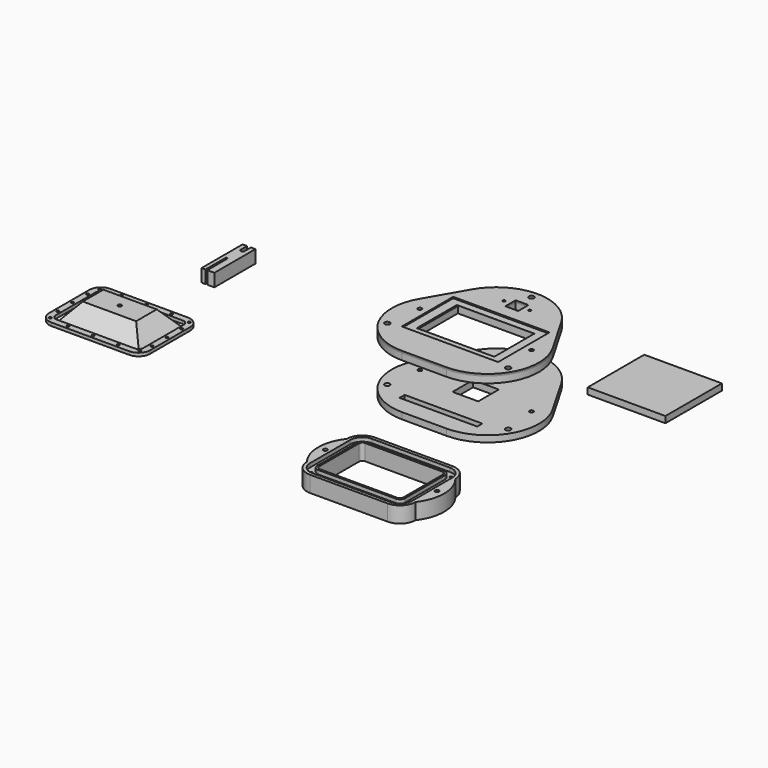
from build123d import *

# Parameters (mm, degrees)
F0_R            = 4
F0_R_2          = 3
F0_W            = 150
F0_H            = 100
F0_R_3          = 2
F0_W_2          = 20
F0_H_2          = 20
F0_W_3          = 1.5
F0_H_3          = 78
F1_DEPTH        = 10
F2_DEPTH        = 1
F3_START        = 1
F3_DEPTH        = 2
F0_W_4          = 121
F0_H_4          = 110
F4_DEPTH        = 10
F6_DEPTH        = 25
F7_DEPTH        = 6
F8_D            = 4
F9_DEPTH        = 5
F10_D           = 4
F10_CSINK_D     = 8
F10_CSINK_ANGLE = 90
F11_DEPTH       = 25
F0_W_5          = 118
F12_DEPTH       = 10
F14_W           = 40
F14_H           = 40
F14_W_2         = 121
F14_H_2         = 10
F15_DEPTH       = 25
F0_W_6          = 125
F0_H_5          = 82
F16_DEPTH       = 25
F16_TAPER       = 40
F18_D           = 6
F18_DEPTH       = 10
F18_TIP         = 1.8025818571
F19_DEPTH       = 20


with BuildPart() as f1:
    # F0 (on Top) → F1 (new body)
    with BuildSketch(Plane.XY):
        with BuildLine():
            Line((-34.6410161514, -100), (34.6410161514, -100))
            ThreePointArc((34.6410161514, -100), (103.9230484541, -60), (103.9230484541, 20))
            Line((103.9230484541, 20), (69.2820323028, 80))
            ThreePointArc((69.2820323028, 80), (0, 120), (-69.2820323028, 80))
            Line((-69.2820323028, 80), (-103.9230484541, 20))
            ThreePointArc((-103.9230484541, 20), (-103.9230484541, -60), (-34.6410161514, -100))
        make_face()
        with Locations((-94.1006406596, -54.3290302157)):
            Circle(F0_R, mode=Mode.SUBTRACT)
        with Locations((-87, 0)):
            Circle(F0_R_2, mode=Mode.SUBTRACT)
        with Locations((94.1006406596, -54.3290302157)):
            Circle(F0_R, mode=Mode.SUBTRACT)
        Rectangle(F0_W, F0_H, mode=Mode.SUBTRACT)
        with Locations((87, 0)):
            Circle(F0_R_2, mode=Mode.SUBTRACT)
        with Locations((-20, 80.2838653326)):
            Circle(F0_R_3, mode=Mode.SUBTRACT)
        with Locations((0, 80.2838653326)):
            Rectangle(F0_W_2, F0_H_2, mode=Mode.SUBTRACT)
        with Locations((20, 80.2838653326)):
            Circle(F0_R_3, mode=Mode.SUBTRACT)
        with Locations((0, 108.6580604315)):
            Circle(F0_R, mode=Mode.SUBTRACT)
        Rectangle(F0_W, F0_H)
        Polygon((-60.5, -39), (-60.5, 39), (-59, 39), (59, 39), (60.5, 39), (60.5, -39), (59, -39), (-59, -39), align=None, mode=Mode.SUBTRACT)
        with Locations((-59.75, 0)):
            Rectangle(F0_W_3, F0_H_3)
        with Locations((59.75, 0)):
            Rectangle(F0_W_3, F0_H_3)
    extrude(amount=-F1_DEPTH)

    # F5 (on face) → F11 (cut)
    with BuildSketch(Plane(origin=(0, 0, -10), x_dir=(1, 0, 0), z_dir=(0, 0, -1))):
        Polygon((60.5, 62.5), (60.5, 72.5), (-60.5, 72.5), (-60.5, 62.5), (-60.5, 39), (-59, 39), (59, 39), (60.5, 39), align=None)
    extrude(amount=-F11_DEPTH, mode=Mode.SUBTRACT)


with BuildPart() as f2:
    # F0 (on Top) → F2 (new body)
    with BuildSketch(Plane.XY):
        with BuildLine():
            Line((-34.6410161514, -100), (34.6410161514, -100))
            ThreePointArc((34.6410161514, -100), (103.9230484541, -60), (103.9230484541, 20))
            Line((103.9230484541, 20), (69.2820323028, 80))
            ThreePointArc((69.2820323028, 80), (0, 120), (-69.2820323028, 80))
            Line((-69.2820323028, 80), (-103.9230484541, 20))
            ThreePointArc((-103.9230484541, 20), (-103.9230484541, -60), (-34.6410161514, -100))
        make_face()
        with Locations((-94.1006406596, -54.3290302157)):
            Circle(F0_R, mode=Mode.SUBTRACT)
        with Locations((-87, 0)):
            Circle(F0_R_2, mode=Mode.SUBTRACT)
        with Locations((94.1006406596, -54.3290302157)):
            Circle(F0_R, mode=Mode.SUBTRACT)
        Rectangle(F0_W, F0_H, mode=Mode.SUBTRACT)
        with Locations((87, 0)):
            Circle(F0_R_2, mode=Mode.SUBTRACT)
        with Locations((-20, 80.2838653326)):
            Circle(F0_R_3, mode=Mode.SUBTRACT)
        with Locations((0, 80.2838653326)):
            Rectangle(F0_W_2, F0_H_2, mode=Mode.SUBTRACT)
        with Locations((20, 80.2838653326)):
            Circle(F0_R_3, mode=Mode.SUBTRACT)
        with Locations((0, 108.6580604315)):
            Circle(F0_R, mode=Mode.SUBTRACT)
        Rectangle(F0_W, F0_H)
        Polygon((-60.5, -39), (-60.5, 39), (-59, 39), (59, 39), (60.5, 39), (60.5, -39), (59, -39), (-59, -39), align=None, mode=Mode.SUBTRACT)
    extrude(amount=F2_DEPTH)


with BuildPart() as f3:
    # F0 (on Top) → F3 (new body)
    with BuildSketch(Plane.XY.offset(F3_START)):
        with BuildLine():
            Line((-34.6410161514, -100), (34.6410161514, -100))
            ThreePointArc((34.6410161514, -100), (103.9230484541, -60), (103.9230484541, 20))
            Line((103.9230484541, 20), (69.2820323028, 80))
            ThreePointArc((69.2820323028, 80), (0, 120), (-69.2820323028, 80))
            Line((-69.2820323028, 80), (-103.9230484541, 20))
            ThreePointArc((-103.9230484541, 20), (-103.9230484541, -60), (-34.6410161514, -100))
        make_face()
        with Locations((-94.1006406596, -54.3290302157)):
            Circle(F0_R, mode=Mode.SUBTRACT)
        with Locations((-87, 0)):
            Circle(F0_R_2, mode=Mode.SUBTRACT)
        with Locations((94.1006406596, -54.3290302157)):
            Circle(F0_R, mode=Mode.SUBTRACT)
        Rectangle(F0_W, F0_H, mode=Mode.SUBTRACT)
        with Locations((87, 0)):
            Circle(F0_R_2, mode=Mode.SUBTRACT)
        with Locations((-20, 80.2838653326)):
            Circle(F0_R_3, mode=Mode.SUBTRACT)
        with Locations((0, 80.2838653326)):
            Rectangle(F0_W_2, F0_H_2, mode=Mode.SUBTRACT)
        with Locations((20, 80.2838653326)):
            Circle(F0_R_3, mode=Mode.SUBTRACT)
        with Locations((0, 108.6580604315)):
            Circle(F0_R, mode=Mode.SUBTRACT)
    extrude(amount=F3_DEPTH)


with BuildPart() as f4:
    # F0 (on Top) → F4 (new body)
    with BuildSketch(Plane.XY):
        with Locations((270.5340873003, 10.6164294481)):
            Rectangle(F0_W_4, F0_H_4)
    extrude(amount=F4_DEPTH)


with BuildPart() as f6:
    # F0 (on Top) → F6 (new body)
    with BuildSketch(Plane.XY):
        with BuildLine():
            ThreePointArc((223.1106657982, -358.8882369786), (222.6106657982, -357.2299245834), (223.1106657982, -355.5716121883))
            Line((223.1106657982, -355.5716121883), (223.1106657982, -318.2299245834))
            ThreePointArc((223.1106657982, -318.2299245834), (216.0812285467, -301.259361835), (199.1106657982, -294.2299245834))
            Line((199.1106657982, -294.2299245834), (78.1106657982, -294.2299245834))
            ThreePointArc((78.1106657982, -294.2299245834), (61.1401030497, -301.259361835), (54.1106657982, -318.2299245834))
            Line((54.1106657982, -318.2299245834), (54.1106657982, -355.5716121883))
            ThreePointArc((54.1106657982, -355.5716121883), (54.4829471215, -356.3638991797), (54.6106657982, -357.2299245834))
            ThreePointArc((54.6106657982, -357.2299245834), (54.4829471215, -358.0959499872), (54.1106657982, -358.8882369786))
            Line((54.1106657982, -358.8882369786), (54.1106657982, -396.2299245834))
            ThreePointArc((54.1106657982, -396.2299245834), (61.1401030497, -413.2004873319), (78.1106657982, -420.2299245834))
            Line((78.1106657982, -420.2299245834), (199.1106657982, -420.2299245834))
            ThreePointArc((199.1106657982, -420.2299245834), (216.0812285467, -413.2004873319), (223.1106657982, -396.2299245834))
            Line((223.1106657982, -396.2299245834), (223.1106657982, -358.8882369786))
        make_face()
        with BuildLine():
            ThreePointArc((59.1106657982, -318.2299245834), (64.6756369556, -304.7948957409), (78.1106657982, -299.2299245834))
            Line((78.1106657982, -299.2299245834), (199.1106657982, -299.2299245834))
            ThreePointArc((199.1106657982, -299.2299245834), (212.5456946407, -304.7948957409), (218.1106657982, -318.2299245834))
            Line((218.1106657982, -318.2299245834), (218.1106657982, -396.2299245834))
            ThreePointArc((218.1106657982, -396.2299245834), (212.5456946407, -409.664953426), (199.1106657982, -415.2299245834))
            Line((199.1106657982, -415.2299245834), (78.1106657982, -415.2299245834))
            ThreePointArc((78.1106657982, -415.2299245834), (64.6756369556, -409.664953426), (59.1106657982, -396.2299245834))
            Line((59.1106657982, -396.2299245834), (59.1106657982, -318.2299245834))
        make_face(mode=Mode.SUBTRACT)
        with BuildLine():
            Line((199.1106657982, -299.2299245834), (78.1106657982, -299.2299245834))
            ThreePointArc((78.1106657982, -299.2299245834), (64.6756369556, -304.7948957409), (59.1106657982, -318.2299245834))
            Line((59.1106657982, -318.2299245834), (59.1106657982, -396.2299245834))
            ThreePointArc((59.1106657982, -396.2299245834), (64.6756369556, -409.664953426), (78.1106657982, -415.2299245834))
            Line((78.1106657982, -415.2299245834), (199.1106657982, -415.2299245834))
            ThreePointArc((199.1106657982, -415.2299245834), (212.5456946407, -409.664953426), (218.1106657982, -396.2299245834))
            Line((218.1106657982, -396.2299245834), (218.1106657982, -318.2299245834))
            ThreePointArc((218.1106657982, -318.2299245834), (212.5456946407, -304.7948957409), (199.1106657982, -299.2299245834))
        make_face()
        with BuildLine():
            ThreePointArc((70.1106657982, -318.2299245834), (72.4538115487, -312.5730703339), (78.1106657982, -310.2299245834))
            Line((78.1106657982, -310.2299245834), (199.1106657982, -310.2299245834))
            ThreePointArc((199.1106657982, -310.2299245834), (204.7675200477, -312.5730703339), (207.1106657982, -318.2299245834))
            Line((207.1106657982, -318.2299245834), (207.1106657982, -396.2299245834))
            ThreePointArc((207.1106657982, -396.2299245834), (204.7675200477, -401.8867788329), (199.1106657982, -404.2299245834))
            Line((199.1106657982, -404.2299245834), (78.1106657982, -404.2299245834))
            ThreePointArc((78.1106657982, -404.2299245834), (72.4538115487, -401.8867788329), (70.1106657982, -396.2299245834))
            Line((70.1106657982, -396.2299245834), (70.1106657982, -318.2299245834))
        make_face(mode=Mode.SUBTRACT)
        with BuildLine():
            Line((199.1106657982, -310.2299245834), (78.1106657982, -310.2299245834))
            ThreePointArc((78.1106657982, -310.2299245834), (72.4538115487, -312.5730703339), (70.1106657982, -318.2299245834))
            Line((70.1106657982, -318.2299245834), (70.1106657982, -396.2299245834))
            ThreePointArc((70.1106657982, -396.2299245834), (72.4538115487, -401.8867788329), (78.1106657982, -404.2299245834))
            Line((78.1106657982, -404.2299245834), (199.1106657982, -404.2299245834))
            ThreePointArc((199.1106657982, -404.2299245834), (204.7675200477, -401.8867788329), (207.1106657982, -396.2299245834))
            Line((207.1106657982, -396.2299245834), (207.1106657982, -318.2299245834))
            ThreePointArc((207.1106657982, -318.2299245834), (204.7675200477, -312.5730703339), (199.1106657982, -310.2299245834))
        make_face()
        with BuildLine():
            ThreePointArc((73.1106657982, -318.2299245834), (74.5751318923, -314.6943906775), (78.1106657982, -313.2299245834))
            Line((78.1106657982, -313.2299245834), (199.1106657982, -313.2299245834))
            ThreePointArc((199.1106657982, -313.2299245834), (202.6461997041, -314.6943906775), (204.1106657982, -318.2299245834))
            Line((204.1106657982, -318.2299245834), (204.1106657982, -396.2299245834))
            ThreePointArc((204.1106657982, -396.2299245834), (202.6461997041, -399.7654584894), (199.1106657982, -401.2299245834))
            Line((199.1106657982, -401.2299245834), (78.1106657982, -401.2299245834))
            ThreePointArc((78.1106657982, -401.2299245834), (74.5751318923, -399.7654584894), (73.1106657982, -396.2299245834))
            Line((73.1106657982, -396.2299245834), (73.1106657982, -318.2299245834))
        make_face(mode=Mode.SUBTRACT)
        with BuildLine():
            Line((54.1106657982, -355.5716121883), (54.1106657982, -318.2299245834))
            ThreePointArc((54.1106657982, -318.2299245834), (40.659391154, -357.2299245834), (54.1106657982, -396.2299245834))
            Line((54.1106657982, -396.2299245834), (54.1106657982, -358.8882369786))
            ThreePointArc((54.1106657982, -358.8882369786), (48.6106657982, -357.2299245834), (54.1106657982, -355.5716121883))
        make_face()
        with BuildLine():
            ThreePointArc((223.1106657982, -355.5716121883), (226.476691202, -354.3576432602), (228.6106657982, -357.2299245834))
            ThreePointArc((228.6106657982, -357.2299245834), (226.476691202, -360.1022059067), (223.1106657982, -358.8882369786))
            Line((223.1106657982, -358.8882369786), (223.1106657982, -396.2299245834))
            ThreePointArc((223.1106657982, -396.2299245834), (236.5619404423, -357.2299245834), (223.1106657982, -318.2299245834))
            Line((223.1106657982, -318.2299245834), (223.1106657982, -355.5716121883))
        make_face()
    extrude(amount=-F6_DEPTH)

    # F0 (on Top) → F7 (cut)
    with BuildSketch(Plane.XY):
        with BuildLine():
            Line((199.1106657982, -299.2299245834), (78.1106657982, -299.2299245834))
            ThreePointArc((78.1106657982, -299.2299245834), (64.6756369556, -304.7948957409), (59.1106657982, -318.2299245834))
            Line((59.1106657982, -318.2299245834), (59.1106657982, -396.2299245834))
            ThreePointArc((59.1106657982, -396.2299245834), (64.6756369556, -409.664953426), (78.1106657982, -415.2299245834))
            Line((78.1106657982, -415.2299245834), (199.1106657982, -415.2299245834))
            ThreePointArc((199.1106657982, -415.2299245834), (212.5456946407, -409.664953426), (218.1106657982, -396.2299245834))
            Line((218.1106657982, -396.2299245834), (218.1106657982, -318.2299245834))
            ThreePointArc((218.1106657982, -318.2299245834), (212.5456946407, -304.7948957409), (199.1106657982, -299.2299245834))
        make_face()
        with BuildLine():
            ThreePointArc((70.1106657982, -318.2299245834), (72.4538115487, -312.5730703339), (78.1106657982, -310.2299245834))
            Line((78.1106657982, -310.2299245834), (199.1106657982, -310.2299245834))
            ThreePointArc((199.1106657982, -310.2299245834), (204.7675200477, -312.5730703339), (207.1106657982, -318.2299245834))
            Line((207.1106657982, -318.2299245834), (207.1106657982, -396.2299245834))
            ThreePointArc((207.1106657982, -396.2299245834), (204.7675200477, -401.8867788329), (199.1106657982, -404.2299245834))
            Line((199.1106657982, -404.2299245834), (78.1106657982, -404.2299245834))
            ThreePointArc((78.1106657982, -404.2299245834), (72.4538115487, -401.8867788329), (70.1106657982, -396.2299245834))
            Line((70.1106657982, -396.2299245834), (70.1106657982, -318.2299245834))
        make_face(mode=Mode.SUBTRACT)
    extrude(amount=-F7_DEPTH, mode=Mode.SUBTRACT)

    # F8 (through all)
    with Locations(Plane.XY):
        with Locations((68.5647242522, -308.6839830374), (99.5444750786, -304.7299245834), (138.6106657982, -304.7299245834), (177.6768565178, -304.7299245834), (208.6566073442, -308.6839830374), (212.6106657982, -328.3349871635), (212.6106657982, -357.2299245834), (212.6106657982, -386.1248620033), (208.6566073442, -405.7758661295), (177.6768565178, -409.7299245834), (138.6106657982, -409.7299245834), (99.5444750786, -409.7299245834), (68.5647242522, -405.7758661295), (64.6106657982, -386.1248620033), (64.6106657982, -328.3349871635)):
            Hole(F8_D / 2)


with BuildPart() as f9:
    # F0 (on Top) → F9 (new body)
    with BuildSketch(Plane.XY):
        with BuildLine():
            Line((-290.5930222716, -197.0301026583), (-411.5930222716, -197.0301026583))
            ThreePointArc((-411.5930222716, -197.0301026583), (-424.3209443329, -202.3021805969), (-429.5930222716, -215.0301026583))
            Line((-429.5930222716, -215.0301026583), (-429.5930222716, -293.0301026583))
            ThreePointArc((-429.5930222716, -293.0301026583), (-424.3209443329, -305.7580247196), (-411.5930222716, -311.0301026583))
            Line((-411.5930222716, -311.0301026583), (-290.5930222716, -311.0301026583))
            ThreePointArc((-290.5930222716, -311.0301026583), (-277.8651002102, -305.7580247196), (-272.5930222716, -293.0301026583))
            Line((-272.5930222716, -293.0301026583), (-272.5930222716, -215.0301026583))
            ThreePointArc((-272.5930222716, -215.0301026583), (-277.8651002102, -202.3021805969), (-290.5930222716, -197.0301026583))
        make_face()
        with BuildLine():
            ThreePointArc((-419.5930222716, -215.0301026583), (-417.2498765211, -209.3732484088), (-411.5930222716, -207.0301026583))
            Line((-411.5930222716, -207.0301026583), (-290.5930222716, -207.0301026583))
            ThreePointArc((-290.5930222716, -207.0301026583), (-284.9361680221, -209.3732484088), (-282.5930222716, -215.0301026583))
            Line((-282.5930222716, -215.0301026583), (-282.5930222716, -293.0301026583))
            ThreePointArc((-282.5930222716, -293.0301026583), (-284.9361680221, -298.6869569078), (-290.5930222716, -301.0301026583))
            Line((-290.5930222716, -301.0301026583), (-411.5930222716, -301.0301026583))
            ThreePointArc((-411.5930222716, -301.0301026583), (-417.2498765211, -298.6869569078), (-419.5930222716, -293.0301026583))
            Line((-419.5930222716, -293.0301026583), (-419.5930222716, -215.0301026583))
        make_face(mode=Mode.SUBTRACT)
    extrude(amount=F9_DEPTH)

    # F10 (through all)
    with Locations(Plane(origin=(0, 0, 0), x_dir=(1, 0, 0), z_dir=(0, 0, -1))):
        with Locations((-420.785410427, 205.8377145028), (-390.1592129912, 202.0301026583), (-351.0930222716, 202.0301026583), (-424.5930222716, 225.1351652384), (-424.5930222716, 254.0301026583), (-424.5930222716, 282.9250400782), (-420.785410427, 302.2224908137), (-390.1592129912, 306.0301026583), (-351.0930222716, 306.0301026583), (-312.026831552, 306.0301026583), (-281.4006341162, 302.2224908137), (-277.5930222716, 282.9250400782), (-277.5930222716, 254.0301026583), (-277.5930222716, 225.1351652384), (-281.4006341162, 205.8377145028), (-312.026831552, 202.0301026583)):
            CounterSinkHole(F10_D / 2, F10_CSINK_D / 2, counter_sink_angle=F10_CSINK_ANGLE)


with BuildPart() as f12:
    # F0 (on Top) → F12 (new body)
    with BuildSketch(Plane.XY):
        with BuildLine():
            Line((-34.6410161514, -100), (34.6410161514, -100))
            ThreePointArc((34.6410161514, -100), (103.9230484541, -60), (103.9230484541, 20))
            Line((103.9230484541, 20), (69.2820323028, 80))
            ThreePointArc((69.2820323028, 80), (0, 120), (-69.2820323028, 80))
            Line((-69.2820323028, 80), (-103.9230484541, 20))
            ThreePointArc((-103.9230484541, 20), (-103.9230484541, -60), (-34.6410161514, -100))
        make_face()
        with Locations((-94.1006406596, -54.3290302157)):
            Circle(F0_R, mode=Mode.SUBTRACT)
        with Locations((-87, 0)):
            Circle(F0_R_2, mode=Mode.SUBTRACT)
        with Locations((94.1006406596, -54.3290302157)):
            Circle(F0_R, mode=Mode.SUBTRACT)
        Rectangle(F0_W, F0_H, mode=Mode.SUBTRACT)
        with Locations((87, 0)):
            Circle(F0_R_2, mode=Mode.SUBTRACT)
        with Locations((-20, 80.2838653326)):
            Circle(F0_R_3, mode=Mode.SUBTRACT)
        with Locations((0, 80.2838653326)):
            Rectangle(F0_W_2, F0_H_2, mode=Mode.SUBTRACT)
        with Locations((20, 80.2838653326)):
            Circle(F0_R_3, mode=Mode.SUBTRACT)
        with Locations((0, 108.6580604315)):
            Circle(F0_R, mode=Mode.SUBTRACT)
        Rectangle(F0_W, F0_H)
        Polygon((-60.5, -39), (-60.5, 39), (-59, 39), (59, 39), (60.5, 39), (60.5, -39), (59, -39), (-59, -39), align=None, mode=Mode.SUBTRACT)
        Rectangle(F0_W_5, F0_H_3)
        with Locations((59.75, 0)):
            Rectangle(F0_W_3, F0_H_3)
        with Locations((-59.75, 0)):
            Rectangle(F0_W_3, F0_H_3)
    extrude(amount=F12_DEPTH)


with BuildPart() as f12_1:
    # F13: moved
    add(f12.part.moved(Location((0, 0, -91))))

    # F14 (on face) → F15 (cut)
    with BuildSketch(Plane(origin=(0, 0, -91), x_dir=(1, 0, 0), z_dir=(0, 0, -1))):
        Rectangle(F14_W, F14_H)
        with Locations((0, 67.5)):
            Rectangle(F14_W_2, F14_H_2)
    extrude(amount=-F15_DEPTH, mode=Mode.SUBTRACT)


with BuildPart() as f16:
    # F0 (on Top) → F16 (new body)
    with BuildSketch(Plane.XY):
        with Locations((-351.0930222716, -254.0301026583)):
            Rectangle(F0_W_6, F0_H_5)
    extrude(amount=F16_DEPTH, taper=F16_TAPER)

    # F18
    with Locations(Plane.XY.offset(25)):
        with Locations((-351.0930222716, -254.0301026583)):
            Hole(F18_D / 2, depth=F18_DEPTH)
            with Locations((0, 0, -(F18_DEPTH + F18_TIP / 2))):  # 118° drill point
                Cone(0, F18_D / 2, F18_TIP, mode=Mode.SUBTRACT)


with BuildPart() as f19:
    # F0 (on Top) → F19 (new body)
    with BuildSketch(Plane.XY):
        with BuildLine():
            Line((-340.9322500229, -27.5354653597), (-340.9322500229, -107.5354653597))
            Line((-340.9322500229, -107.5354653597), (-334.8987400532, -107.5354653597))
            Line((-334.8987400532, -107.5354653597), (-334.8987400532, -67.5354653597))
            Line((-334.8987400532, -67.5354653597), (-331.8987400532, -67.5354653597))
            Line((-331.8987400532, -67.5354653597), (-331.8987400532, -107.5354653597))
            Line((-331.8987400532, -107.5354653597), (-320.9322500229, -107.5354653597))
            Line((-320.9322500229, -107.5354653597), (-320.9322500229, -27.5354653597))
            Line((-320.9322500229, -27.5354653597), (-327.9322500229, -27.5354653597))
            ThreePointArc((-327.9322500229, -27.5354653597), (-327.9427584545, -27.7863441405), (-327.9742101313, -28.0354653597))
            ThreePointArc((-327.9742101313, -28.0354653597), (-327.9427584545, -28.2845865788), (-327.9322500229, -28.5354653597))
            ThreePointArc((-327.9322500229, -28.5354653597), (-327.9427584545, -28.7863441405), (-327.9742101313, -29.0354653597))
            ThreePointArc((-327.9742101313, -29.0354653597), (-327.9427584545, -29.2845865788), (-327.9322500229, -29.5354653597))
            ThreePointArc((-327.9322500229, -29.5354653597), (-327.9427584545, -29.7863441405), (-327.9742101313, -30.0354653597))
            ThreePointArc((-327.9742101313, -30.0354653597), (-327.9427584545, -30.2845865788), (-327.9322500229, -30.5354653597))
            ThreePointArc((-327.9322500229, -30.5354653597), (-327.9427584545, -30.7863441405), (-327.9742101313, -31.0354653597))
            ThreePointArc((-327.9742101313, -31.0354653597), (-327.9427584545, -31.2845865788), (-327.9322500229, -31.5354653597))
            ThreePointArc((-327.9322500229, -31.5354653597), (-327.9427584545, -31.7863441405), (-327.9742101313, -32.0354653597))
            ThreePointArc((-327.9742101313, -32.0354653597), (-327.9427584545, -32.2845865788), (-327.9322500229, -32.5354653597))
            ThreePointArc((-327.9322500229, -32.5354653597), (-327.9427584545, -32.7863441405), (-327.9742101313, -33.0354653597))
            ThreePointArc((-327.9742101313, -33.0354653597), (-327.9427584545, -33.2845865788), (-327.9322500229, -33.5354653597))
            ThreePointArc((-327.9322500229, -33.5354653597), (-327.9427584545, -33.7863441405), (-327.9742101313, -34.0354653597))
            ThreePointArc((-327.9742101313, -34.0354653597), (-327.9427584545, -34.2845865788), (-327.9322500229, -34.5354653597))
            ThreePointArc((-327.9322500229, -34.5354653597), (-327.9427584545, -34.7863441405), (-327.9742101313, -35.0354653597))
            ThreePointArc((-327.9742101313, -35.0354653597), (-327.9427584545, -35.2845865788), (-327.9322500229, -35.5354653597))
            ThreePointArc((-327.9322500229, -35.5354653597), (-327.9427584545, -35.7863441405), (-327.9742101313, -36.0354653597))
            ThreePointArc((-327.9742101313, -36.0354653597), (-327.9427584545, -36.2845865788), (-327.9322500229, -36.5354653597))
            ThreePointArc((-327.9322500229, -36.5354653597), (-327.9427584545, -36.7863441405), (-327.9742101313, -37.0354653597))
            ThreePointArc((-327.9742101313, -37.0354653597), (-327.9427584545, -37.2845865788), (-327.9322500229, -37.5354653597))
            ThreePointArc((-327.9322500229, -37.5354653597), (-327.9427584545, -37.7863441405), (-327.9742101313, -38.0354653597))
            ThreePointArc((-327.9742101313, -38.0354653597), (-327.9427584545, -38.2845865788), (-327.9322500229, -38.5354653597))
            ThreePointArc((-327.9322500229, -38.5354653597), (-327.9427584545, -38.7863441405), (-327.9742101313, -39.0354653597))
            ThreePointArc((-327.9742101313, -39.0354653597), (-327.9427584545, -39.2845865788), (-327.9322500229, -39.5354653597))
            ThreePointArc((-327.9322500229, -39.5354653597), (-331.1831288037, -42.5249569281), (-333.8902899144, -39.0354653597))
            ThreePointArc((-333.8902899144, -39.0354653597), (-333.9322500229, -38.5354653597), (-333.8902899144, -38.0354653597))
            ThreePointArc((-333.8902899144, -38.0354653597), (-333.9322500229, -37.5354653597), (-333.8902899144, -37.0354653597))
            ThreePointArc((-333.8902899144, -37.0354653597), (-333.9322500229, -36.5354653597), (-333.8902899144, -36.0354653597))
            ThreePointArc((-333.8902899144, -36.0354653597), (-333.9322500229, -35.5354653597), (-333.8902899144, -35.0354653597))
            ThreePointArc((-333.8902899144, -35.0354653597), (-333.9322500229, -34.5354653597), (-333.8902899144, -34.0354653597))
            ThreePointArc((-333.8902899144, -34.0354653597), (-333.9322500229, -33.5354653597), (-333.8902899144, -33.0354653597))
            ThreePointArc((-333.8902899144, -33.0354653597), (-333.9322500229, -32.5354653597), (-333.8902899144, -32.0354653597))
            ThreePointArc((-333.8902899144, -32.0354653597), (-333.9322500229, -31.5354653597), (-333.8902899144, -31.0354653597))
            ThreePointArc((-333.8902899144, -31.0354653597), (-333.9322500229, -30.5354653597), (-333.8902899144, -30.0354653597))
            ThreePointArc((-333.8902899144, -30.0354653597), (-333.9322500229, -29.5354653597), (-333.8902899144, -29.0354653597))
            ThreePointArc((-333.8902899144, -29.0354653597), (-333.9322500229, -28.5354653597), (-333.8902899144, -28.0354653597))
            ThreePointArc((-333.8902899144, -28.0354653597), (-333.9217415913, -27.7863441405), (-333.9322500229, -27.5354653597))
            Line((-333.9322500229, -27.5354653597), (-340.9322500229, -27.5354653597))
        make_face()
        with BuildLine():
            ThreePointArc((-333.8902899144, -28.5354653597), (-333.9322500229, -28.0354653597), (-333.8902899144, -27.5354653597))
            ThreePointArc((-333.8902899144, -27.5354653597), (-333.9322500229, -27.0354653597), (-333.8902899144, -26.5354653597))
            ThreePointArc((-333.8902899144, -26.5354653597), (-331.1831288037, -23.0459737913), (-327.9322500229, -26.0354653597))
            ThreePointArc((-327.9322500229, -26.0354653597), (-327.9427584545, -26.2863441405), (-327.9742101313, -26.5354653597))
            ThreePointArc((-327.9742101313, -26.5354653597), (-327.9427584545, -26.7845865788), (-327.9322500229, -27.0354653597))
            ThreePointArc((-327.9322500229, -27.0354653597), (-327.9427584545, -27.2863441405), (-327.9742101313, -27.5354653597))
            ThreePointArc((-327.9742101313, -27.5354653597), (-327.9427584545, -27.7845865788), (-327.9322500229, -28.0354653597))
            ThreePointArc((-327.9322500229, -28.0354653597), (-327.9427584545, -28.2863441405), (-327.9742101313, -28.5354653597))
            ThreePointArc((-327.9742101313, -28.5354653597), (-327.9427584545, -28.7845865788), (-327.9322500229, -29.0354653597))
            ThreePointArc((-327.9322500229, -29.0354653597), (-327.9427584545, -29.2863441405), (-327.9742101313, -29.5354653597))
            ThreePointArc((-327.9742101313, -29.5354653597), (-327.9427584545, -29.7845865788), (-327.9322500229, -30.0354653597))
            ThreePointArc((-327.9322500229, -30.0354653597), (-327.9427584545, -30.2863441405), (-327.9742101313, -30.5354653597))
            ThreePointArc((-327.9742101313, -30.5354653597), (-327.9427584545, -30.7845865788), (-327.9322500229, -31.0354653597))
            ThreePointArc((-327.9322500229, -31.0354653597), (-327.9427584545, -31.2863441405), (-327.9742101313, -31.5354653597))
            ThreePointArc((-327.9742101313, -31.5354653597), (-327.9427584545, -31.7845865788), (-327.9322500229, -32.0354653597))
            ThreePointArc((-327.9322500229, -32.0354653597), (-327.9427584545, -32.2863441405), (-327.9742101313, -32.5354653597))
            ThreePointArc((-327.9742101313, -32.5354653597), (-327.9427584545, -32.7845865788), (-327.9322500229, -33.0354653597))
            ThreePointArc((-327.9322500229, -33.0354653597), (-327.9427584545, -33.2863441405), (-327.9742101313, -33.5354653597))
            ThreePointArc((-327.9742101313, -33.5354653597), (-327.9427584545, -33.7845865788), (-327.9322500229, -34.0354653597))
            ThreePointArc((-327.9322500229, -34.0354653597), (-327.9427584545, -34.2863441405), (-327.9742101313, -34.5354653597))
            ThreePointArc((-327.9742101313, -34.5354653597), (-327.9427584545, -34.7845865788), (-327.9322500229, -35.0354653597))
            ThreePointArc((-327.9322500229, -35.0354653597), (-327.9427584545, -35.2863441405), (-327.9742101313, -35.5354653597))
            ThreePointArc((-327.9742101313, -35.5354653597), (-327.9427584545, -35.7845865788), (-327.9322500229, -36.0354653597))
            ThreePointArc((-327.9322500229, -36.0354653597), (-327.9427584545, -36.2863441405), (-327.9742101313, -36.5354653597))
            ThreePointArc((-327.9742101313, -36.5354653597), (-327.9427584545, -36.7845865788), (-327.9322500229, -37.0354653597))
            ThreePointArc((-327.9322500229, -37.0354653597), (-327.9427584545, -37.2863441405), (-327.9742101313, -37.5354653597))
            ThreePointArc((-327.9742101313, -37.5354653597), (-327.9427584545, -37.7845865788), (-327.9322500229, -38.0354653597))
            ThreePointArc((-327.9322500229, -38.0354653597), (-327.9427584545, -38.2863441405), (-327.9742101313, -38.5354653597))
            ThreePointArc((-327.9742101313, -38.5354653597), (-327.9427584545, -38.7845865788), (-327.9322500229, -39.0354653597))
            ThreePointArc((-327.9322500229, -39.0354653597), (-327.9427584545, -39.2863441405), (-327.9742101313, -39.5354653597))
            ThreePointArc((-327.9742101313, -39.5354653597), (-327.9427584545, -39.7845865788), (-327.9322500229, -40.0354653597))
            ThreePointArc((-327.9322500229, -40.0354653597), (-331.1831288037, -43.0249569281), (-333.8902899144, -39.5354653597))
            ThreePointArc((-333.8902899144, -39.5354653597), (-333.9322500229, -39.0354653597), (-333.8902899144, -38.5354653597))
            ThreePointArc((-333.8902899144, -38.5354653597), (-333.9322500229, -38.0354653597), (-333.8902899144, -37.5354653597))
            ThreePointArc((-333.8902899144, -37.5354653597), (-333.9322500229, -37.0354653597), (-333.8902899144, -36.5354653597))
            ThreePointArc((-333.8902899144, -36.5354653597), (-333.9322500229, -36.0354653597), (-333.8902899144, -35.5354653597))
            ThreePointArc((-333.8902899144, -35.5354653597), (-333.9322500229, -35.0354653597), (-333.8902899144, -34.5354653597))
            ThreePointArc((-333.8902899144, -34.5354653597), (-333.9322500229, -34.0354653597), (-333.8902899144, -33.5354653597))
            ThreePointArc((-333.8902899144, -33.5354653597), (-333.9322500229, -33.0354653597), (-333.8902899144, -32.5354653597))
            ThreePointArc((-333.8902899144, -32.5354653597), (-333.9322500229, -32.0354653597), (-333.8902899144, -31.5354653597))
            ThreePointArc((-333.8902899144, -31.5354653597), (-333.9322500229, -31.0354653597), (-333.8902899144, -30.5354653597))
            ThreePointArc((-333.8902899144, -30.5354653597), (-333.9322500229, -30.0354653597), (-333.8902899144, -29.5354653597))
            ThreePointArc((-333.8902899144, -29.5354653597), (-333.9322500229, -29.0354653597), (-333.8902899144, -28.5354653597))
        make_face(mode=Mode.SUBTRACT)
    extrude(amount=F19_DEPTH)


solid = Compound([f1.part, f2.part, f3.part, f4.part, f6.part, f9.part, f12_1.part, f16.part, f19.part])
